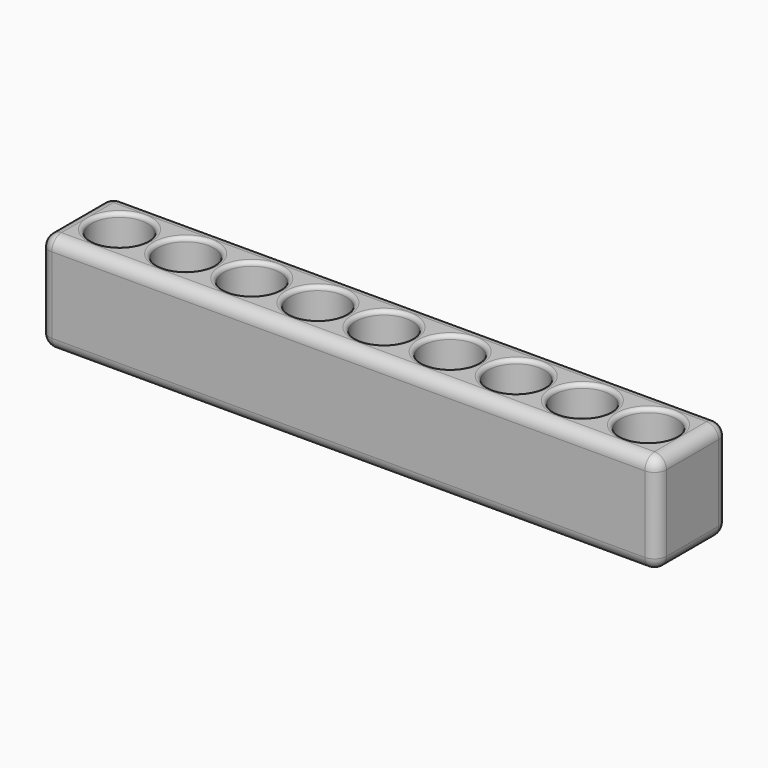
from build123d import *

# Parameters (mm, degrees)
F0_W     = 78.232
F0_H     = 11.3031361252
F0_R     = 3.556
F1_DEPTH = 12.7
F2_DEPTH = 1.27
F3_R     = 1.524
F4_R     = 0.50799


# Not quite as in the source:
# - a fillet or chamfer is up to 0.001 mm smaller than in the source, because OpenCascade refuses the exact size
# - a feature names something its author has since deleted; it is built from what else it names


with BuildPart() as f1:
    # F0 (on Top) → F1 (new body)
    with BuildSketch(Plane.XY):
        with Locations((33.528, 0)):
            Rectangle(F0_W, F0_H)
        Circle(F0_R, mode=Mode.SUBTRACT)
        with Locations((8.382, 0)):
            Circle(F0_R, mode=Mode.SUBTRACT)
        with Locations((16.764, 0)):
            Circle(F0_R, mode=Mode.SUBTRACT)
        with Locations((25.146, 0)):
            Circle(F0_R, mode=Mode.SUBTRACT)
        with Locations((33.528, 0)):
            Circle(F0_R, mode=Mode.SUBTRACT)
        with Locations((41.91, 0)):
            Circle(F0_R, mode=Mode.SUBTRACT)
        with Locations((50.292, 0)):
            Circle(F0_R, mode=Mode.SUBTRACT)
        with Locations((58.674, 0)):
            Circle(F0_R, mode=Mode.SUBTRACT)
        with Locations((67.056, 0)):
            Circle(F0_R, mode=Mode.SUBTRACT)
    extrude(amount=F1_DEPTH)

    # F0 (on Top) → F2 (join)
    with BuildSketch(Plane.XY):
        Circle(F0_R)
        with Locations((8.382, 0)):
            Circle(F0_R)
        with Locations((16.764, 0)):
            Circle(F0_R)
        with Locations((25.146, 0)):
            Circle(F0_R)
        with Locations((33.528, 0)):
            Circle(F0_R)
        with Locations((41.91, 0)):
            Circle(F0_R)
        with Locations((50.292, 0)):
            Circle(F0_R)
        with Locations((58.674, 0)):
            Circle(F0_R)
        with Locations((67.056, 0)):
            Circle(F0_R)
    extrude(amount=F2_DEPTH)

    # F3
    f3_edges = [f1.edges().sort_by_distance(p)[0] for p in [
        (-5.588, -5.651568, 6.35),
        (72.644, -5.651568, 6.35),
        (33.528, -5.651568, 0),
        (33.528, -5.651568, 12.7),
        (-5.588, 5.651568, 6.35),
        (-5.588, 0, 0),
        (-5.588, 0, 12.7),
        (72.644, 5.651568, 6.35),
        (33.528, 5.651568, 0),
        (33.528, 5.651568, 12.7),
        (72.644, 0, 0),
        (72.644, 0, 12.7),
    ]]
    fillet(f3_edges, radius=F3_R)

    # F4 (radius 0.508 in the source; OpenCascade refuses exactly that, so slightly less here)
    f4_edges = [f1.edges().sort_by_distance(p)[0] for p in [
        (-3.556, 0, 12.7),
        (63.5, 0, 12.7),
        (55.118, 0, 12.7),
        (38.354, 0, 12.7),
        (46.736, 0, 12.7),
        (29.972, 0, 12.7),
        (21.59, 0, 12.7),
        (13.208, 0, 12.7),
        (4.826, 0, 12.7),
    ]]
    fillet(f4_edges, radius=F4_R)


solid = f1.part
